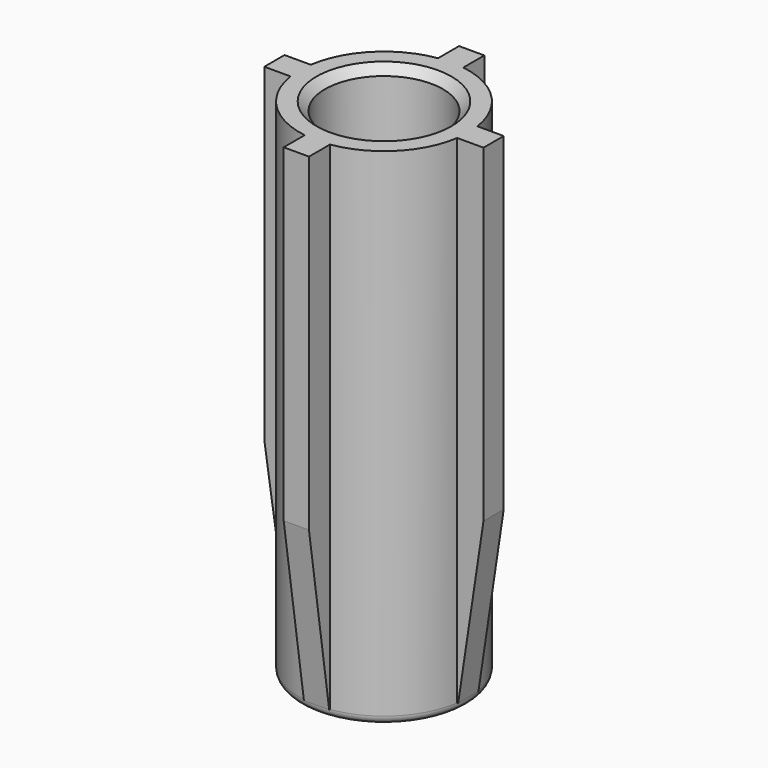
from build123d import *

# Parameters (mm, degrees)
F1_R        = 5
F1_R_2      = 3.5
F2_DEPTH    = 30
F4_W        = 1.5
F4_H        = 2.639524132
F5_DEPTH    = 29.5
F6_COUNT    = 4
F8_R        = 3.5
F8_R_2      = 1.25
F9_DEPTH    = 1.5
F10_SIZE2   = 1.49999
F10_SIZE    = 9.99999
F10_2_SIZE2 = 1.49999
F10_2_SIZE  = 9.99999
F10_3_SIZE2 = 1.49999
F10_3_SIZE  = 9.99999
F10_4_SIZE2 = 1.49999
F10_4_SIZE  = 9.99999
F11_SIZE    = 0.5
F12_R       = 0.49999


# Not quite as in the source:
# - a fillet or chamfer is up to 0.001 mm smaller than in the source, because OpenCascade refuses the exact size


with BuildPart() as f2:
    # F1 (on offset) → F2 (new body)
    with BuildSketch(Plane.XY):
        with Locations((-25, 25)):
            Circle(F1_R)
        with Locations((-25, 25)):
            Circle(F1_R_2, mode=Mode.SUBTRACT)
    extrude(amount=-F2_DEPTH)

    # F4 (on offset) → F5 (join)
    with BuildSketch(Plane.XY):
        with Locations((-25, 30.180237934)):
            Rectangle(F4_W, F4_H)
    extrude(amount=-F5_DEPTH)

    # F6: F2 ×4 about axis
    f6_axis = Axis((-25, 25, 0), (0, 0, 1))


with BuildPart() as f2_1:
    add(f2.part)
    for i in range(1, F6_COUNT):
        add(f2.part.rotate(f6_axis, i * 360 / F6_COUNT))

    # F8 (on offset) → F9 (join)
    with BuildSketch(Plane.XY.offset(-30)):
        with Locations((-25, 25)):
            Circle(F8_R)
        with Locations((-25, 25)):
            Circle(F8_R_2, mode=Mode.SUBTRACT)
    extrude(amount=F9_DEPTH)

    # F10 (size 10 and 1.5 in the source; OpenCascade refuses exactly that, so slightly less here)
    f10_edges = [f2_1.edges().sort_by_distance(p)[0] for p in [
        (-25, 18.5, -29.5),
    ]]
    f10_side = f2_1.faces().sort_by_distance((-25, 18.5, -14.75))[0]
    chamfer(f10_edges, length=F10_SIZE, length2=F10_SIZE2, reference=f10_side)

    # F10#2 (size 10 and 1.5 in the source; OpenCascade refuses exactly that, so slightly less here)
    f10_2_edges = [f2_1.edges().sort_by_distance(p)[0] for p in [
        (-18.5, 25, -29.5),
    ]]
    f10_2_side = f2_1.faces().sort_by_distance((-18.5, 25, -14.75))[0]
    chamfer(f10_2_edges, length=F10_2_SIZE, length2=F10_2_SIZE2, reference=f10_2_side)

    # F10#3 (size 10 and 1.5 in the source; OpenCascade refuses exactly that, so slightly less here)
    f10_3_edges = [f2_1.edges().sort_by_distance(p)[0] for p in [
        (-25, 31.5, -29.5),
    ]]
    f10_3_side = f2_1.faces().sort_by_distance((-25, 31.5, -14.75))[0]
    chamfer(f10_3_edges, length=F10_3_SIZE, length2=F10_3_SIZE2, reference=f10_3_side)

    # F10#4 (size 10 and 1.5 in the source; OpenCascade refuses exactly that, so slightly less here)
    f10_4_edges = [f2_1.edges().sort_by_distance(p)[0] for p in [
        (-31.5, 25, -29.5),
    ]]
    f10_4_side = f2_1.faces().sort_by_distance((-31.5, 25, -14.75))[0]
    chamfer(f10_4_edges, length=F10_4_SIZE, length2=F10_4_SIZE2, reference=f10_4_side)

    # F11
    f11_edges = [f2_1.edges().sort_by_distance(p)[0] for p in [
        (-28.5, 25, 0),
        (-26.25, 25, -28.5),
    ]]
    chamfer(f11_edges, length=F11_SIZE)

    # F12 (radius 0.5 in the source; OpenCascade refuses exactly that, so slightly less here)
    f12_edges = [f2_1.edges().sort_by_distance(p)[0] for p in [
        (-30, 25, -30),
    ]]
    fillet(f12_edges, radius=F12_R)


solid = f2_1.part
